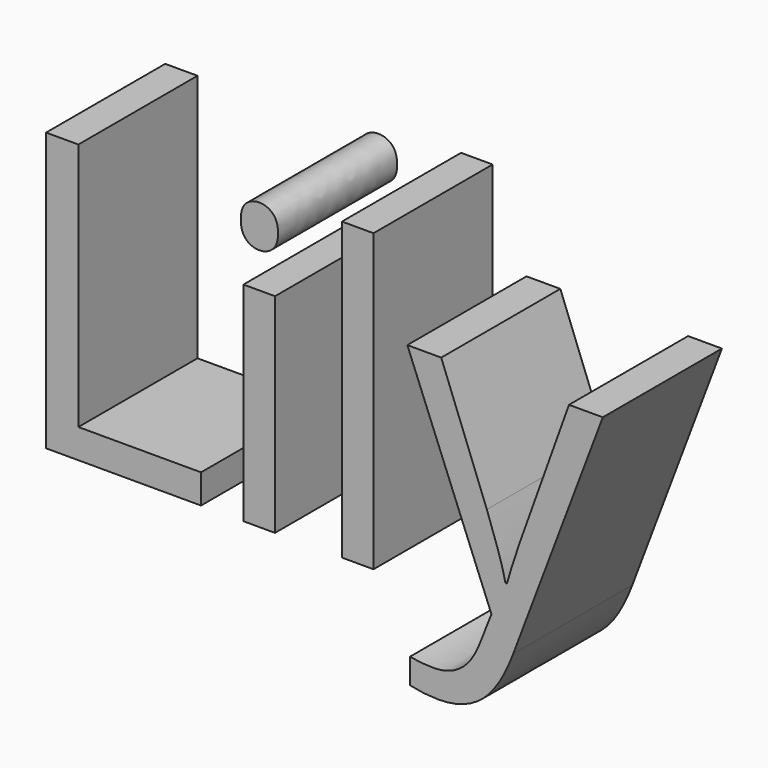
from build123d import *

# Parameters (mm, degrees)
F0_TEXT_SIZE = 66.4253951982
F1_DEPTH     = 25.4


# Not quite as in the source:
# - Text() gives the source's letters only with a copy of the font that has no kerning and outlines rounded to 1/6400 em; it was checked with that copy


with BuildPart() as f1:
    # F0 (on Front) → F1 (new body)
    with BuildSketch(Plane.XZ):
        with Locations((-38.9996916056, -19.7457130998)):
            Text('Lily', F0_TEXT_SIZE, font='Open Sans', text_align=(TextAlign.LEFT, TextAlign.BOTTOM))
    extrude(amount=F1_DEPTH)


solid = f1.part
